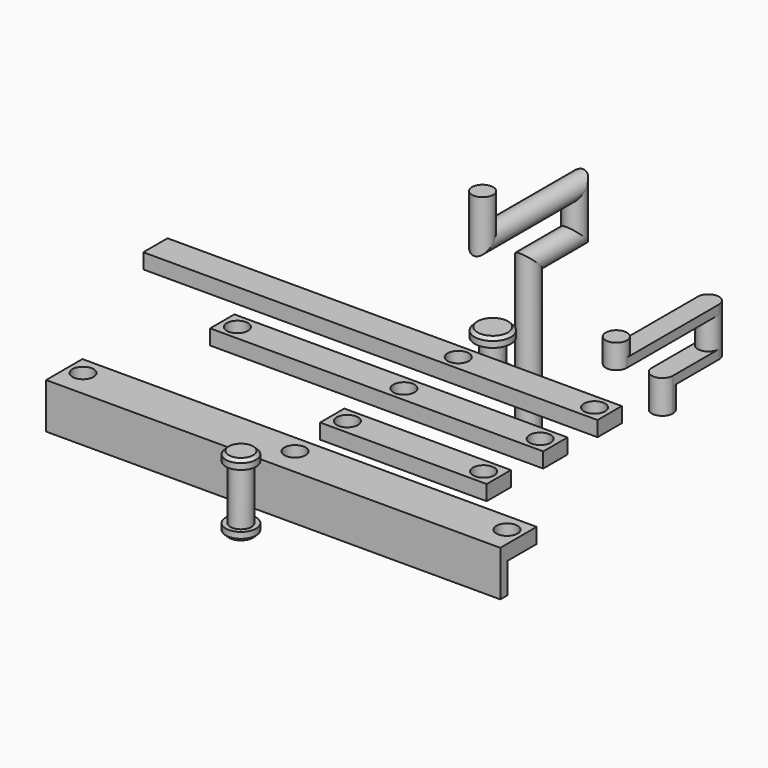
from build123d import *

# Parameters (mm, degrees)
F0_W      = 110
F0_H      = 10
F0_R      = 3.5
F1_DEPTH  = 5
F2_W      = 150
F2_H      = 10
F2_R      = 3.5
F3_DEPTH  = 5
F4_W      = 55
F4_H      = 10
F4_R      = 3.5
F5_DEPTH  = 5
F6_W      = 150
F6_H      = 3
F7_DEPTH  = 10
F6_H_2    = 12
F6_R      = 3.5
F8_DEPTH  = 5
F11_SIZE  = 1
F14_R     = 3.5
F18_SIZE  = 1
F20_DEPTH = 3
F21_DEPTH = 5
F22_DEPTH = 13
F24_DEPTH = 13
F27_DEPTH = 3
F28_DEPTH = 8
F29_DEPTH = 8


# Not quite as in the source:
# - a feature names something its author has since deleted; it is built from what else it names


with BuildPart() as f1:
    # F0 (on Top) → F1 (new body)
    with BuildSketch(Plane.XY):
        with Locations((-5, 0)):
            Rectangle(F0_W, F0_H)
        with Locations((-55, 0)):
            Circle(F0_R, mode=Mode.SUBTRACT)
        Circle(F0_R, mode=Mode.SUBTRACT)
        with Locations((45, 0)):
            Circle(F0_R, mode=Mode.SUBTRACT)
    extrude(amount=F1_DEPTH)


with BuildPart() as f3:
    # F2 (on Top) → F3 (new body)
    with BuildSketch(Plane.XY):
        with Locations((-25, 22.4212598074)):
            Rectangle(F2_W, F2_H)
        with Locations((0, 22.4212598074)):
            Circle(F2_R, mode=Mode.SUBTRACT)
        with Locations((45, 22.4212598074)):
            Circle(F2_R, mode=Mode.SUBTRACT)
    extrude(amount=F3_DEPTH)


with BuildPart() as f5:
    # F4 (on Top) → F5 (new body)
    with BuildSketch(Plane.XY):
        with Locations((22.5, -23.3469191799)):
            Rectangle(F4_W, F4_H)
        with Locations((0, -23.3469191799)):
            Circle(F4_R, mode=Mode.SUBTRACT)
        with Locations((45, -23.3469191799)):
            Circle(F4_R, mode=Mode.SUBTRACT)
    extrude(amount=F5_DEPTH)


with BuildPart() as f7:
    # F6 (on Top) → F7 (new body)
    with BuildSketch(Plane.XY):
        with Locations((0, -52.4558726716)):
            Rectangle(F6_W, F6_H)
    extrude(amount=-F7_DEPTH)

    # F6 (on Top) → F8 (join)
    with BuildSketch(Plane.XY):
        with Locations((0, -44.9558726716)):
            Rectangle(F6_W, F6_H_2)
        with Locations((-70, -44.9558726716)):
            Circle(F6_R, mode=Mode.SUBTRACT)
        with Locations((0, -44.9558726716)):
            Circle(F6_R, mode=Mode.SUBTRACT)
        with Locations((70, -44.9558726716)):
            Circle(F6_R, mode=Mode.SUBTRACT)
        with Locations((0, -52.4558726716)):
            Rectangle(F6_W, F6_H)
    extrude(amount=F8_DEPTH)


with BuildPart() as f10:
    # F9 (on Right) → F10 (revolve)
    with BuildSketch(Plane.YZ):
        Polygon((33.1747402222, -5), (30.6747411754, -5), (30.6747411754, -8), (36.6747402222, -8), (36.6747402222, 8), (30.6747411754, 8), (30.6747411754, 5), (33.1747402222, 5), (33.1747402222, 0), align=None)
    revolve(axis=Axis((0, 36.6747402222, 0.4419543714), (0, 0, 1)))

    # F11
    f11_edges = [f10.edges().sort_by_distance(p)[0] for p in [
        (0, 42.674739, 8),
        (0, 42.674739, -8),
    ]]
    chamfer(f11_edges, length=F11_SIZE)


with BuildPart() as f15:
    # F15: sweep along a path in F12
    with BuildLine(Plane.YZ) as f15_path:
        Line((51.4675094231, -28.7774660638), (51.4675094231, 21.2225339362))
        Line((51.4675094231, 21.2225339362), (70.4675094231, 21.2225339362))
        Line((70.4675094231, 21.2225339362), (70.4675094231, 35.2225339362))
        Line((70.4675094231, 35.2225339362), (32.4675094231, 35.2225339362))
        Line((32.4675094231, 35.2225339362), (32.4675094231, 49.2225339362))
    # F14 (on plane+point) → F15 (sweep)
    with BuildSketch(Plane.XY.offset(-28.7774660638)):
        with Locations((0, 51.4675094231)):
            Circle(F14_R)
    sweep(path=f15_path.line, transition=Transition.RIGHT)


with BuildPart() as f17:
    # F16 (on Right) → F17 (revolve)
    with BuildSketch(Plane.YZ):
        Polygon((-67.2618212021, -9.7663268149), (-67.2618212021, 14.2336731851), (-72.2618212021, 14.2336731851), (-72.2618212021, 11.2336731851), (-70.7618212021, 11.2336731851), (-70.7618212021, 6.2336731851), (-70.7618212021, 3.2336731851), (-70.7618212021, -6.7663268149), (-72.2618212021, -6.7663268149), (-72.2618212021, -9.7663268149), align=None)
    revolve(axis=Axis((0, -67.2618212021, 2.2336731851), (0, 0, -1)))

    # F18
    f18_edges = [f17.edges().sort_by_distance(p)[0] for p in [
        (0, -62.261821, -9.766327),
        (0, -62.261821, 14.233673),
    ]]
    chamfer(f18_edges, length=F18_SIZE)


with BuildPart() as f20:
    # F19 (on Top) → F20 (new body)
    with BuildSketch(Plane.XY):
        with BuildLine():
            ThreePointArc((40.3348876363, 51.5639246599), (43.9828572132, 48.3937493663), (47.3196705598, 51.8899430275))
            ThreePointArc((47.3196705598, 51.8899430275), (43.9828572132, 55.3861366886), (40.3348876363, 52.215961395))
            Line((40.3348876363, 52.215961395), (40.3348876363, 51.5639246599))
        make_face()
        with BuildLine():
            ThreePointArc((40.3348876363, 52.215961395), (43.9828572132, 55.3861366886), (47.3196705598, 51.8899430275))
            Line((47.3196705598, 51.8899430275), (47.3196705598, 70.8899430275))
            ThreePointArc((47.3196705598, 70.8899430275), (43.9828572132, 67.3937493663), (40.3348876363, 70.5639246599))
            Line((40.3348876363, 70.5639246599), (40.3348876363, 52.215961395))
        make_face()
        with BuildLine():
            ThreePointArc((40.3348876363, 70.5639246599), (43.9828572132, 67.3937493663), (47.3196705598, 70.8899430275))
            ThreePointArc((47.3196705598, 70.8899430275), (43.6564839064, 74.3861366886), (40.3348876363, 70.5639246599))
        make_face()
    extrude(amount=F20_DEPTH)

    # F19 (on Top) → F24 (join)
    with BuildSketch(Plane.XY):
        with BuildLine():
            ThreePointArc((40.3348876363, 70.5639246599), (43.9828572132, 67.3937493663), (47.3196705598, 70.8899430275))
            ThreePointArc((47.3196705598, 70.8899430275), (43.6564839064, 74.3861366886), (40.3348876363, 70.5639246599))
        make_face()
    extrude(amount=F24_DEPTH)

    # F26 (on offset) → F27 (join)
    with BuildSketch(Plane.XY.offset(13)):
        with BuildLine():
            ThreePointArc((40.3348876363, 70.5639246599), (43.9828572132, 67.3937493663), (47.3196705598, 70.8899430275))
            ThreePointArc((47.3196705598, 70.8899430275), (43.6564839064, 74.3861366886), (40.3348876363, 70.5639246599))
        make_face()
        with BuildLine():
            ThreePointArc((40.3348876363, 52.215961395), (43.9828572132, 55.3861366886), (47.3196705598, 51.8899430275))
            Line((47.3196705598, 51.8899430275), (47.3196705598, 70.8899430275))
            ThreePointArc((47.3196705598, 70.8899430275), (43.9828572132, 67.3937493663), (40.3348876363, 70.5639246599))
            Line((40.3348876363, 70.5639246599), (40.3348876363, 52.215961395))
        make_face()
        with BuildLine():
            ThreePointArc((40.3348876363, 51.5639246599), (43.9828572132, 48.3937493663), (47.3196705598, 51.8899430275))
            ThreePointArc((47.3196705598, 51.8899430275), (43.9828572132, 55.3861366886), (40.3348876363, 52.215961395))
            Line((40.3348876363, 52.215961395), (40.3348876363, 51.5639246599))
        make_face()
        with BuildLine():
            ThreePointArc((40.3348876363, 33.215961395), (43.9828572132, 36.3861366886), (47.3196705598, 32.8899430275))
            Line((47.3196705598, 32.8899430275), (47.3196705598, 51.8899430275))
            ThreePointArc((47.3196705598, 51.8899430275), (43.9828572132, 48.3937493663), (40.3348876363, 51.5639246599))
            Line((40.3348876363, 51.5639246599), (40.3348876363, 33.215961395))
        make_face()
        with BuildLine():
            Line((40.3348876363, 33.215961395), (40.3348876363, 32.5639246599))
            ThreePointArc((40.3348876363, 32.5639246599), (43.9828572132, 29.3937493663), (47.3196705598, 32.8899430275))
            ThreePointArc((47.3196705598, 32.8899430275), (43.9828572132, 36.3861366886), (40.3348876363, 33.215961395))
        make_face()
    extrude(amount=F27_DEPTH)

    # F26 (on offset) → F28 (join)
    with BuildSketch(Plane.XY.offset(13)):
        with BuildLine():
            Line((40.3348876363, 33.215961395), (40.3348876363, 32.5639246599))
            ThreePointArc((40.3348876363, 32.5639246599), (43.9828572132, 29.3937493663), (47.3196705598, 32.8899430275))
            ThreePointArc((47.3196705598, 32.8899430275), (43.9828572132, 36.3861366886), (40.3348876363, 33.215961395))
        make_face()
    extrude(amount=F28_DEPTH)

    # F19 (on Top) → F29 (join)
    with BuildSketch(Plane.XY):
        with BuildLine():
            ThreePointArc((40.3348876363, 51.5639246599), (43.9828572132, 48.3937493663), (47.3196705598, 51.8899430275))
            ThreePointArc((47.3196705598, 51.8899430275), (43.9828572132, 55.3861366886), (40.3348876363, 52.215961395))
            Line((40.3348876363, 52.215961395), (40.3348876363, 51.5639246599))
        make_face()
    extrude(amount=-F29_DEPTH)


with BuildPart() as f21:
    # F19 (on Top) → F21 (new body)
    with BuildSketch(Plane.XY):
        with BuildLine():
            ThreePointArc((40.3348876363, 51.5639246599), (43.9828572132, 48.3937493663), (47.3196705598, 51.8899430275))
            ThreePointArc((47.3196705598, 51.8899430275), (43.9828572132, 55.3861366886), (40.3348876363, 52.215961395))
            Line((40.3348876363, 52.215961395), (40.3348876363, 51.5639246599))
        make_face()
    extrude(amount=-F21_DEPTH)


with BuildPart() as f22:
    # F19 (on Top) → F22 (new body)
    with BuildSketch(Plane.XY):
        with BuildLine():
            ThreePointArc((40.3348876363, 70.5639246599), (43.9828572132, 67.3937493663), (47.3196705598, 70.8899430275))
            ThreePointArc((47.3196705598, 70.8899430275), (43.6564839064, 74.3861366886), (40.3348876363, 70.5639246599))
        make_face()
    extrude(amount=F22_DEPTH)


solid = Compound([f1.part, f3.part, f5.part, f7.part, f10.part, f15.part, f17.part, f20.part])
